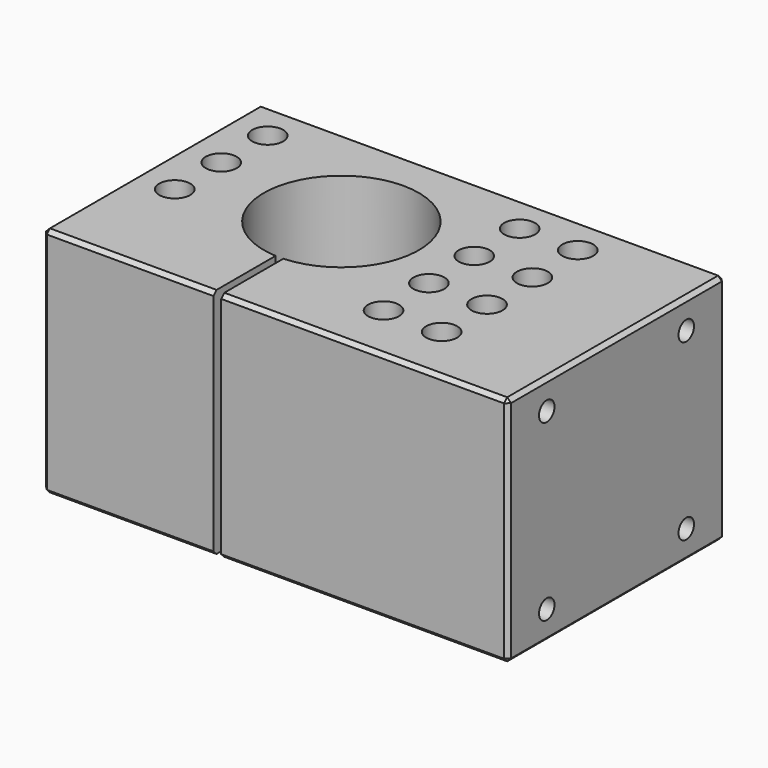
from build123d import *

# Parameters (mm, degrees)
F1_DEPTH       = 60
F3_D           = 5
F3_DEPTH       = 65
F3_CBORE_D     = 12
F3_CBORE_DEPTH = 25
F3_TIP         = 1.5021515476
F4_SIZE        = 1
F6_D           = 5
F6_DEPTH       = 23.5
F6_TIP         = 1.5021515476
F9_D           = 8
F9_ON_F7_D     = 8


with BuildPart() as f1:
    # F0 (on Top) → F1 (new body)
    with BuildSketch(Plane.XY):
        with BuildLine():
            Line((60, 35), (-60, 35))
            Line((-60, 35), (-60, -35))
            Line((-60, -35), (-16, -35))
            Line((-16, -35), (-16, -14.9749843554))
            ThreePointArc((-16, -14.9749843554), (-15, 25), (-14, -14.9749843554))
            Line((-14, -14.9749843554), (-14, -35))
            Line((-14, -35), (60, -35))
            Line((60, -35), (60, 35))
        make_face()
    extrude(amount=-F1_DEPTH)

    # F3
    with Locations(Plane(origin=(-60, 0, 0), x_dir=(0, -1, 0), z_dir=(-1, 0, 0))):
        with Locations((25, -45), (25, -15)):
            CounterBoreHole(F3_D / 2, F3_CBORE_D / 2, F3_CBORE_DEPTH, depth=F3_DEPTH)
            with Locations((0, 0, -(F3_DEPTH + F3_TIP / 2))):  # 118° drill point
                Cone(0, F3_D / 2, F3_TIP, mode=Mode.SUBTRACT)

    # F4
    f4_edges = [f1.edges().sort_by_distance(p)[0] for p in [
        (-60, -35, -30),
        (-60, 35, -30),
        (60, -35, -30),
        (60, 35, -30),
        (0, 35, -60),
        (-60, 0, -60),
        (-38, -35, -60),
        (23, -35, -60),
        (60, 0, -60),
        (-60, 0, 0),
        (-38, -35, 0),
        (23, -35, 0),
        (60, 0, 0),
        (0, 35, 0),
    ]]
    chamfer(f4_edges, length=F4_SIZE)

    # F6
    with Locations(Plane.YZ.offset(60)):
        with Locations((-22.5, -7.5), (22.5, -7.5), (22.5, -52.5), (-22.5, -52.5)):
            Hole(F6_D / 2, depth=F6_DEPTH)
            with Locations((0, 0, -(F6_DEPTH + F6_TIP / 2))):  # 118° drill point
                Cone(0, F6_D / 2, F6_TIP, mode=Mode.SUBTRACT)

    # F9 (through all)
    with Locations(Plane(origin=(0, 0, -60), x_dir=(1, 0, 0), z_dir=(0, 0, -1))):
        with Locations((15, -25), (15.2912072429, -10.0028269883), (15.5824144859, 4.9943460233), (15.8736217288, 19.991519035), (30.8736217288, 19.991519035), (30.5824144859, 4.9943460233), (30.2912072429, -10.0028269883), (30, -25)):
            Hole(F9_D / 2)

    # F9 on F7 (through all)
    with Locations(Plane(origin=(0, 0, -60), x_dir=(1, 0, 0), z_dir=(0, 0, -1))):
        with Locations((-50, -25), (-50, -10), (-50, 5)):
            Hole(F9_ON_F7_D / 2)


solid = f1.part
